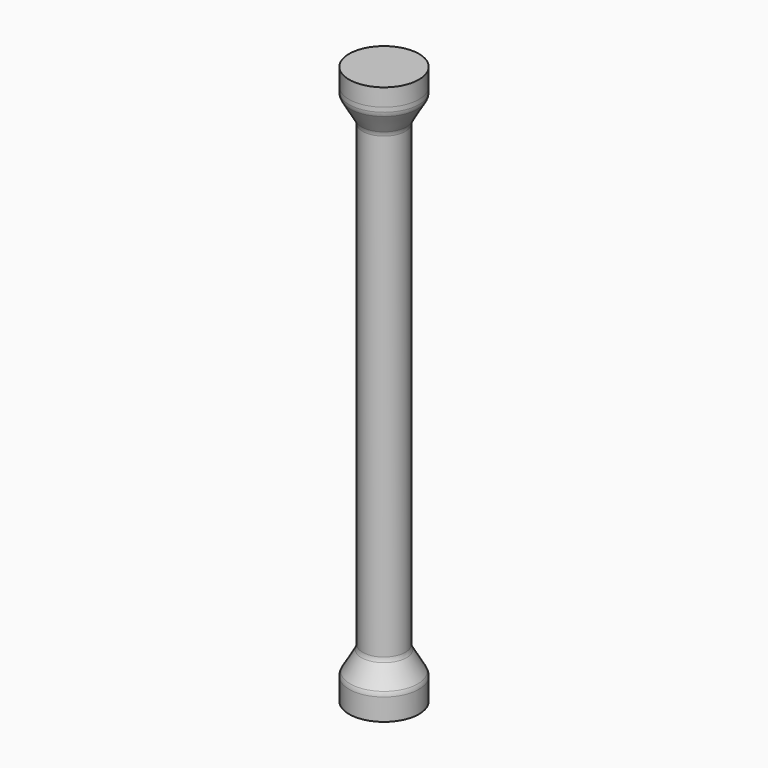
from build123d import *

# Parameters (mm, degrees)
F0_W        = 4.9
F0_H        = 60
F2_S5_R     = 8
F2_T6_DEPTH = 15
F3_S5_R     = 8
F3_T6_DEPTH = 15
F4_R        = 2


# Not quite as in the source:
# - a fillet or chamfer that OpenCascade refuses, or shapes differently, is made with other operations: its cross-section is extruded or revolved along the edge and cut away or added


with BuildPart() as f1:
    # F0 (on Front) → F1 (revolve)
    with BuildSketch(Plane.XZ):
        Polygon((0, 64), (0, 60), (4.9, 60), (8, 60), (8, 64), align=None)
        with Locations((2.45, 30)):
            Rectangle(F0_W, F0_H)
        with Locations((2.45, -30)):
            Rectangle(F0_W, F0_H)
        Polygon((4.9, -60), (0, -60), (0, -64), (8, -64), (8, -60), align=None)
    revolve(axis=Axis((0, 0, -30), (0, 0, -1)))

    # F2: chamfer of 4 x 6.9282032303 on 1 edges, made by hand


with BuildPart() as f2_tool2:
    # F2_s3 → F2_t4 (revolve)
    with BuildSketch(Plane.XZ):
        Polygon((4.9, 53.0717967697), (8.9, 60), (4.9, 60), align=None)
    revolve(axis=Axis((0, 0, 60), (0, 0, -1)))

    # F2_s5 → F2_t6 (intersect, symmetric)
    with BuildSketch(Plane.XY.offset(56.5)):
        Circle(F2_S5_R)
    extrude(amount=F2_T6_DEPTH, both=True, mode=Mode.INTERSECT)


with BuildPart() as f1_1:
    add(f1.part)

    # F2_t1: union F2_tool2
    add(f2_tool2.part)

    # F3: chamfer of 4 x 6.9282032303 on 1 edges, made by hand


with BuildPart() as f3_tool2:
    # F3_s3 → F3_t4 (revolve)
    with BuildSketch(Plane.XZ):
        Polygon((8.9, -60), (4.9, -53.0717967697), (4.9, -60), align=None)
    revolve(axis=Axis((0, 0, -60), (0, 0, -1)))

    # F3_s5 → F3_t6 (intersect, symmetric)
    with BuildSketch(Plane.XY.offset(-56.5)):
        Circle(F3_S5_R)
    extrude(amount=F3_T6_DEPTH, both=True, mode=Mode.INTERSECT)


with BuildPart() as f1_2:
    add(f1_1.part)

    # F3_t1: union F3_tool2
    add(f3_tool2.part)

    # F4
    f4_edges = [f1_2.edges().sort_by_distance(p)[0] for p in [
        (-8, 0, -58.441154),
        (-4.9, 0, -53.071797),
        (-4.9, 0, 53.071797),
        (-8, 0, 58.441154),
    ]]
    fillet(f4_edges, radius=F4_R)


solid = f1_2.part
